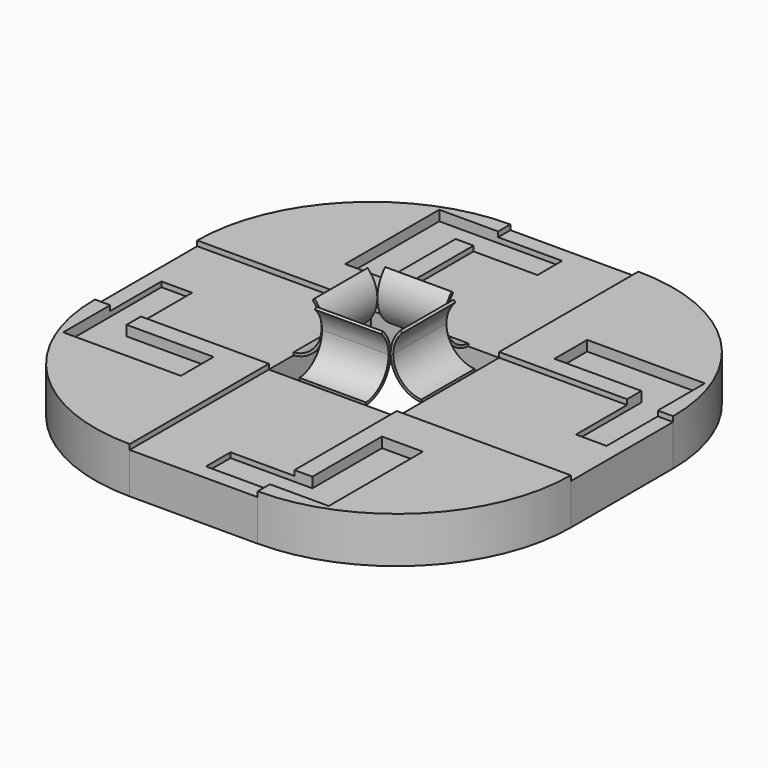
from build123d import *

# Parameters (mm, degrees)
F0_W            = 34
F0_H            = 25
F0_W_2          = 25
F0_H_2          = 34
F1_DEPTH        = 9
F2_W            = 34
F2_H            = 25
F2_W_2          = 25
F2_H_2          = 34
F3_DEPTH        = 1
F5_DEPTH        = 6.5
F5_COPIES_COUNT = 4
F7_W            = 6
F7_H            = 3.5
F7_H_2          = 12.5
F8_DEPTH        = 2
F8_COPIES_COUNT = 4


# Not quite as in the source:
# - a pattern or mirror of a feature is missing from the dataset's text; its kind, count and spacing are read off the source's solid


with BuildPart() as f1:
    # F0 (on Top) → F1 (new body)
    with BuildSketch(Plane.XY):
        with Locations((-29.5, 0)):
            Rectangle(F0_W, F0_H)
        with Locations((0, -29.5)):
            Rectangle(F0_W_2, F0_H_2)
        with Locations((29.5, 0)):
            Rectangle(F0_W, F0_H)
        with Locations((0, 29.5)):
            Rectangle(F0_W_2, F0_H_2)
        with BuildLine():
            Line((-12.5, 12.5), (-12.5, 46.5))
            ThreePointArc((-12.5, 46.5), (-36.5416305603, 36.5416305603), (-46.5, 12.5))
            Line((-46.5, 12.5), (-12.5, 12.5))
        make_face()
        with BuildLine():
            ThreePointArc((46.5, 12.5), (36.5416305603, 36.5416305603), (12.5, 46.5))
            Line((12.5, 46.5), (12.5, 12.5))
            Line((12.5, 12.5), (46.5, 12.5))
        make_face()
        with BuildLine():
            Line((46.5, -12.5), (12.5, -12.5))
            Line((12.5, -12.5), (12.5, -46.5))
            ThreePointArc((12.5, -46.5), (36.5416305603, -36.5416305603), (46.5, -12.5))
        make_face()
        with BuildLine():
            Line((-12.5, -46.5), (-12.5, -12.5))
            Line((-12.5, -12.5), (-46.5, -12.5))
            ThreePointArc((-46.5, -12.5), (-36.5416305603, -36.5416305603), (-12.5, -46.5))
        make_face()
    extrude(amount=F1_DEPTH)

    # F2 (on face) → F3 (cut)
    with BuildSketch(Plane.XY.offset(9)):
        with Locations((-29.5, 0)):
            Rectangle(F2_W, F2_H)
        with Locations((0, -29.5)):
            Rectangle(F2_W_2, F2_H_2)
        with Locations((29.5, 0)):
            Rectangle(F2_W, F2_H)
        with Locations((0, 29.5)):
            Rectangle(F2_W_2, F2_H_2)
    extrude(amount=-F3_DEPTH, mode=Mode.SUBTRACT)

    # F7 (on face) → F8 (cut)
    with BuildSketch(Plane.XY.offset(9)):
        with Locations((40.5, 14.25)):
            Rectangle(F7_W, F7_H)
        with Locations((40.5, 6.25)):
            Rectangle(F7_W, F7_H_2)
        Polygon((20.5, 16), (37.5, 16), (43.5, 16), (43.5, 24), (20.5, 24), align=None)
    f8 = extrude(amount=-F8_DEPTH, mode=Mode.SUBTRACT)

    # F8_copies: F8 ×4 about axis
    f8_copies_axis = Axis((0, 0, 0), (0, 0, 1))
    for i in range(1, F8_COPIES_COUNT):
        add(f8.rotate(f8_copies_axis, i * 360 / F8_COPIES_COUNT), mode=Mode.SUBTRACT)


with BuildPart() as f5:
    # F4 (on Front) → F5 (new body, symmetric)
    with BuildSketch(Plane.XZ):
        with BuildLine():
            Line((-12.5, 8.5), (-12.5, 8.0192593016))
            ThreePointArc((-12.5, 8.0192593016), (-8.2303039929, 10.0841195668), (-6.5, 14.5))
            ThreePointArc((-6.5, 14.5), (-6.9947830387, 16.9874423104), (-8.4038059223, 19.0961940777))
            Line((-8.4038059223, 19.0961940777), (-8.7573593129, 18.7426406871))
            ThreePointArc((-8.7573593129, 18.7426406871), (-7.4567228049, 16.7961005942), (-7, 14.5))
            ThreePointArc((-7, 14.5), (-8.5841195668, 10.4379807977), (-12.5, 8.5208696284))
            Line((-12.5, 8.5208696284), (-12.5, 8.5))
        make_face()
    extrude(amount=F5_DEPTH, both=True)


with BuildPart() as f5_copies_1:
    # F5_copies: instance of F5
    add(f5.part.rotate(Axis((0, 0, 0), (0, 0, 1)), 1 * 360 / F5_COPIES_COUNT))


with BuildPart() as f5_copies_2:
    # F5_copies: instance of F5
    add(f5.part.rotate(Axis((0, 0, 0), (0, 0, 1)), 2 * 360 / F5_COPIES_COUNT))


with BuildPart() as f5_copies_3:
    # F5_copies: instance of F5
    add(f5.part.rotate(Axis((0, 0, 0), (0, 0, 1)), 3 * 360 / F5_COPIES_COUNT))


solid = Compound([f1.part, f5.part, f5_copies_1.part, f5_copies_2.part, f5_copies_3.part])
